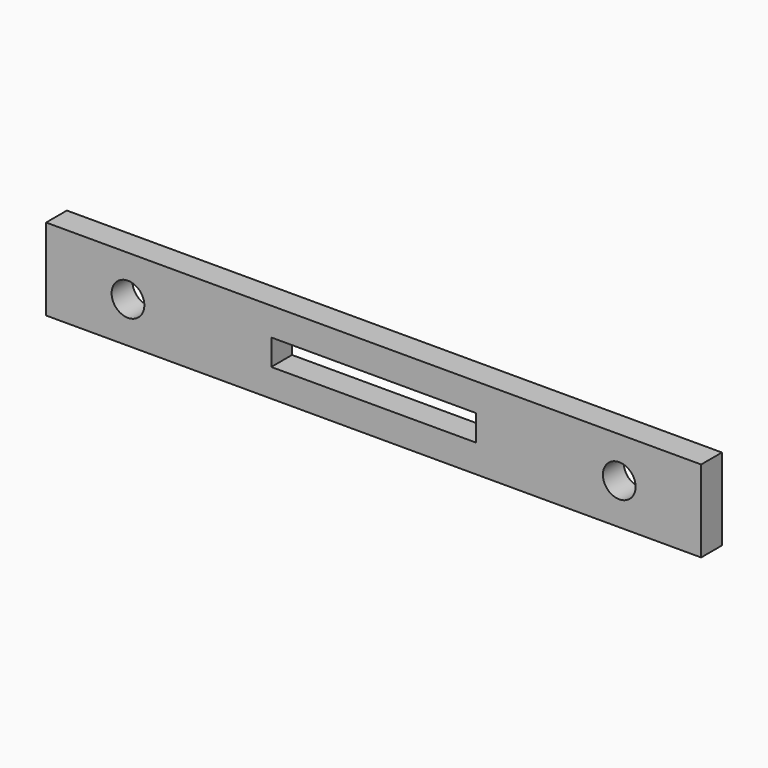
from build123d import *

# Parameters (mm, degrees)
F0_W     = 160
F0_H     = 20
F0_R     = 4
F0_W_2   = 50
F0_H_2   = 6.35
F1_DEPTH = 6.35


# Not quite as in the source:
# - a length typed as a fraction of an inch, garbled in the dataset ("3 / 203.2 mm" for 3/8 in), is restored


with BuildPart() as f1:
    # F0 (on Front) → F1 (new body)
    with BuildSketch(Plane.XZ):
        Rectangle(F0_W, F0_H)
        with Locations((-60, 0)):
            Circle(F0_R, mode=Mode.SUBTRACT)
        Rectangle(F0_W_2, F0_H_2, mode=Mode.SUBTRACT)
        with Locations((60, 0)):
            Circle(F0_R, mode=Mode.SUBTRACT)
    extrude(amount=F1_DEPTH)


solid = f1.part
